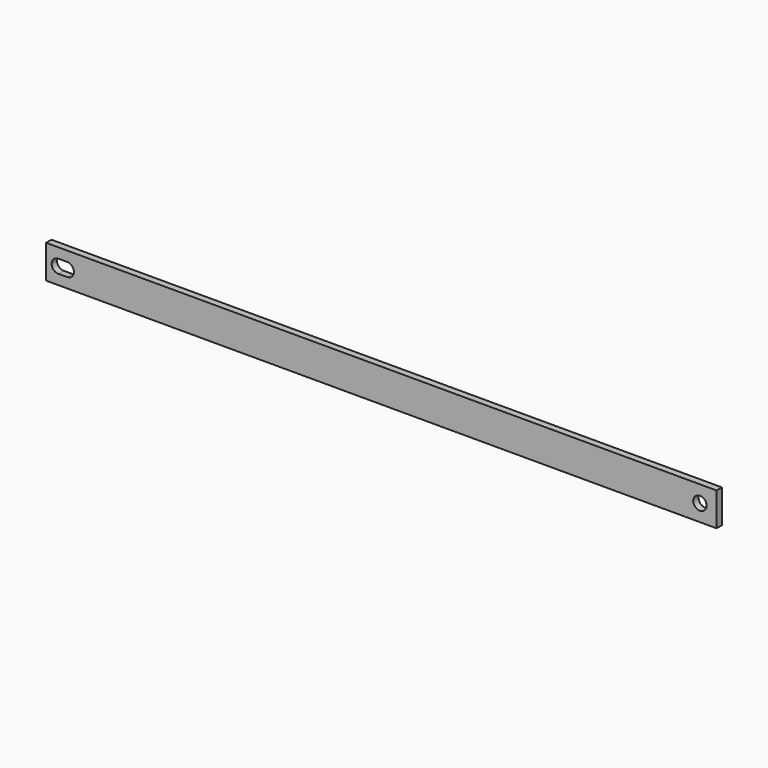
from build123d import *

# Parameters (mm, degrees)
F0_W     = 100.5
F0_H     = 5
F0_R     = 1
F1_DEPTH = 1
F2_W     = 3.3293967307
F2_H     = 2
F3_DEPTH = 25
F4_R     = 0.99999


# Not quite as in the source:
# - a fillet or chamfer is up to 0.001 mm smaller than in the source, because OpenCascade refuses the exact size


with BuildPart() as f1:
    # F0 (on Front) → F1 (new body)
    with BuildSketch(Plane.XZ):
        Rectangle(F0_W, F0_H)
        with Locations((-47.75, 0)):
            Circle(F0_R, mode=Mode.SUBTRACT)
        with Locations((47.75, 0)):
            Circle(F0_R, mode=Mode.SUBTRACT)
    extrude(amount=F1_DEPTH)

    # F2 (on face) → F3 (cut)
    with BuildSketch(Plane.XZ.offset(1)):
        with Locations((-47.75, 0)):
            Rectangle(F2_W, F2_H)
    extrude(amount=-F3_DEPTH, mode=Mode.SUBTRACT)

    # F4 (radius 1 in the source; OpenCascade refuses exactly that, so slightly less here)
    f4_edges = [f1.edges().sort_by_distance(p)[0] for p in [
        (-46.085302, -0.5, 1),
        (-46.085302, -0.5, -1),
        (-49.414698, -0.5, 1),
        (-49.414698, -0.5, -1),
    ]]
    fillet(f4_edges, radius=F4_R)


solid = f1.part
